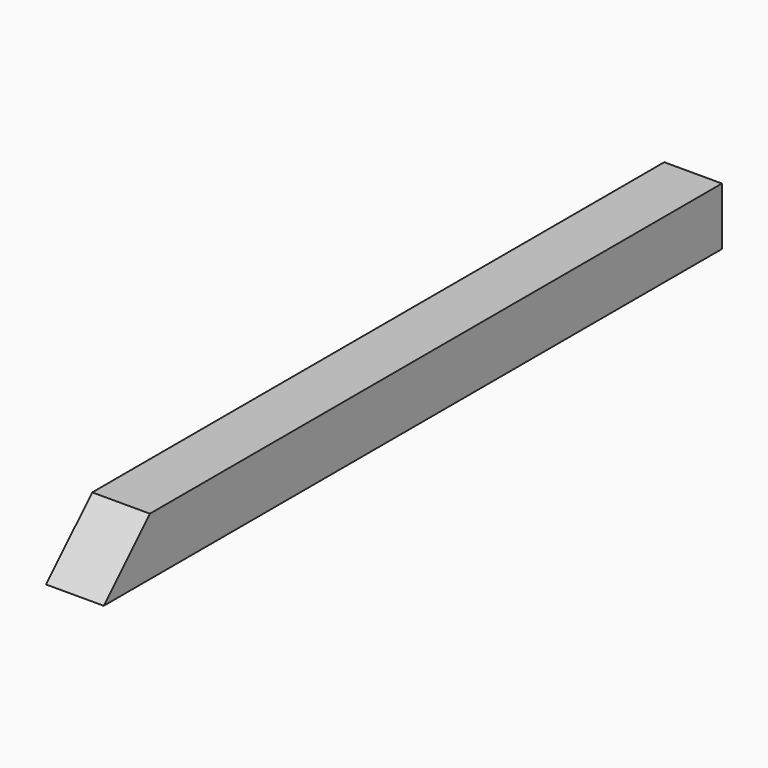
from build123d import *

# Parameters (mm, degrees)
F0_W     = 10
F0_H     = 10
F1_DEPTH = 134
F2_SIZE  = 9.99999


# Not quite as in the source:
# - a fillet or chamfer is up to 0.001 mm smaller than in the source, because OpenCascade refuses the exact size


with BuildPart() as f1:
    # F0 (on Front) → F1 (new body)
    with BuildSketch(Plane.XZ):
        Rectangle(F0_W, F0_H)
    extrude(amount=F1_DEPTH)

    # F2 (size 10 in the source; OpenCascade refuses exactly that, so slightly less here)
    f2_edges = [f1.edges().sort_by_distance(p)[0] for p in [
        (0, -134, 5),
    ]]
    chamfer(f2_edges, length=F2_SIZE)


solid = f1.part
